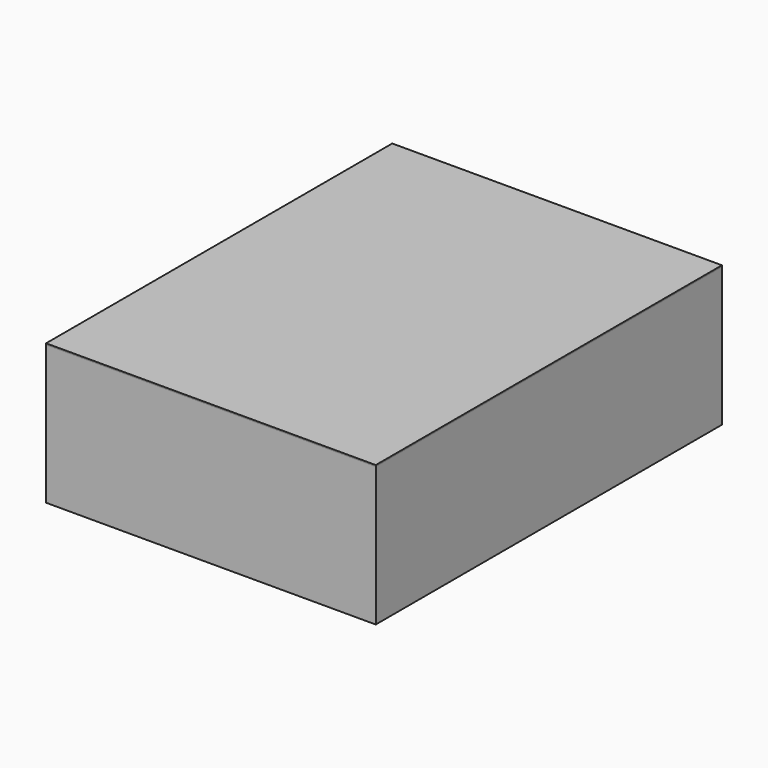
from build123d import *

# Parameters (mm, degrees)
F0_W     = 25.4
F0_H     = 10.715625
F1_DEPTH = 33.3375
F2_W     = 25.4
F2_H     = 0.1016
F3_DEPTH = 33.3375


# Not quite as in the source:
# - a feature names something its author has since deleted; it is built from what else it names


with BuildPart() as f1:
    # F0 (on Front) → F1 (new body)
    with BuildSketch(Plane.XZ):
        with Locations((12.7, 5.3578125)):
            Rectangle(F0_W, F0_H)
    extrude(amount=F1_DEPTH)


with BuildPart() as f3:
    # F2 (on Front) → F3 (new body)
    with BuildSketch(Plane.XZ):
        with Locations((12.7, 10.766425)):
            Rectangle(F2_W, F2_H)
    extrude(amount=F3_DEPTH)


solid = Compound([f1.part, f3.part])
